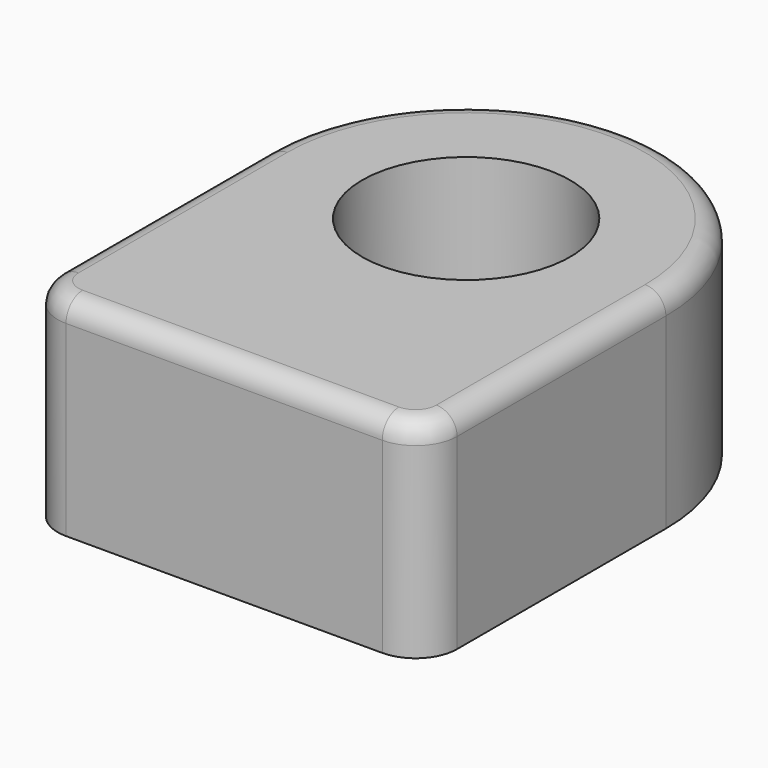
from build123d import *

# Parameters (mm, degrees)
F1_DEPTH    = 25.4
F3_D        = 25.4
F4_R        = 2.54
F5_T1_DEPTH = 38.1
F5_T4_ANGLE = 90
F5_T6_ANGLE = 90


# Not quite as in the source:
# - a fillet or chamfer that OpenCascade refuses, or shapes differently, is made with other operations: its cross-section is extruded or revolved along the edge and cut away or added


with BuildPart() as f1:
    # F0 (on Top) → F1 (new body)
    with BuildSketch(Plane.XY):
        with BuildLine():
            Line((0, 36.9386635721), (0, 0))
            Line((0, 0), (48.7761497498, 0))
            Line((48.7761497498, 0), (48.7761497498, 36.9386635721))
            ThreePointArc((48.7761497498, 36.9386635721), (24.3880748749, 61.326738447), (0, 36.9386635721))
        make_face()
    extrude(amount=F1_DEPTH)

    # F3 (through all)
    with Locations(Plane.XY.offset(25.4)):
        with Locations((24.3880748749, 36.9386635721)):
            Hole(F3_D / 2)

    # F4
    f4_edges = [f1.edges().sort_by_distance(p)[0] for p in [
        (24.388075, 0, 25.4),
        (48.77615, 18.469332, 25.4),
    ]]
    fillet(f4_edges, radius=F4_R)

    # F5: fillet of radius 5.08 on 2 edges, made by hand

    # F5_s2 → F5_t1 (cut)
    with BuildSketch(Plane.XY.offset(-12.7)):
        with BuildLine():
            ThreePointArc((43.6961497498, 0), (47.2882521982, 1.4878975516), (48.7761497498, 5.08))
            Line((48.7761497498, 5.08), (48.7761497498, 0))
            Line((48.7761497498, 0), (43.6961497498, 0))
        make_face()
        with BuildLine():
            ThreePointArc((0, 5.08), (1.4878975516, 1.4878975516), (5.08, 0))
            Line((5.08, 0), (0, 0))
            Line((0, 0), (0, 5.08))
        make_face()
    extrude(amount=F5_T1_DEPTH, mode=Mode.SUBTRACT)

    # F5_s3 → F5_t4 (revolve, cut)
    with BuildSketch(Plane.XZ.offset(-5.08)):
        with BuildLine():
            ThreePointArc((2.54, 25.4), (0.7439487758, 24.6560512242), (0, 22.86))
            Line((0, 22.86), (0, 25.4))
            Line((0, 25.4), (2.54, 25.4))
        make_face()
    revolve(axis=Axis((5.08, 5.08, 25.4), (0, 0, 1)), revolution_arc=F5_T4_ANGLE, mode=Mode.SUBTRACT)

    # F5_s5 → F5_t6 (revolve, cut)
    with BuildSketch(Plane.YZ.offset(43.6961497498)):
        with BuildLine():
            ThreePointArc((2.54, 25.4), (0.7439487758, 24.6560512242), (0, 22.86))
            Line((0, 22.86), (0, 25.4))
            Line((0, 25.4), (2.54, 25.4))
        make_face()
    revolve(axis=Axis((43.6961497498, 5.08, 25.4), (0, 0, 1)), revolution_arc=F5_T6_ANGLE, mode=Mode.SUBTRACT)


solid = f1.part
